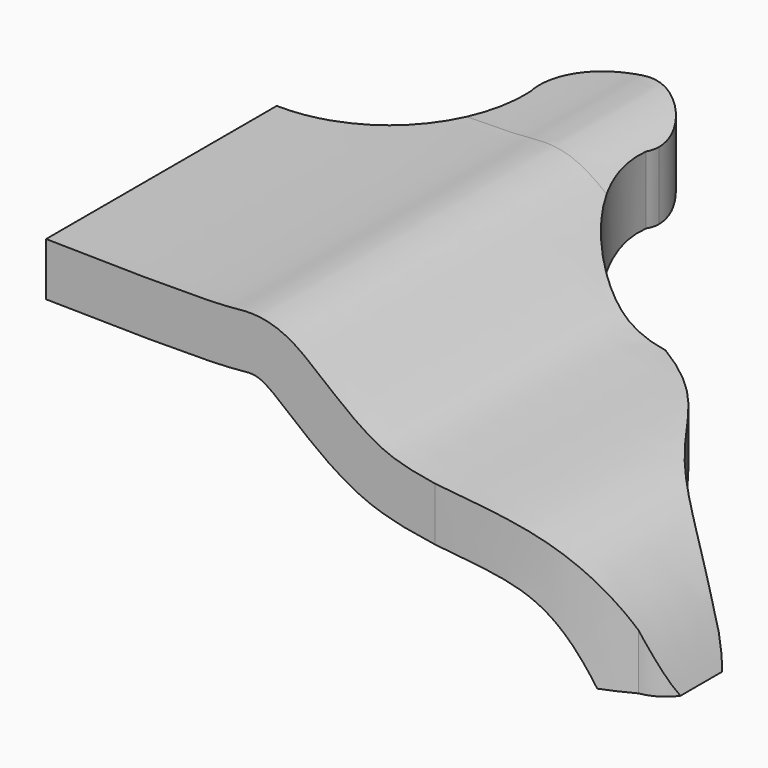
from build123d import *

# Parameters (mm, degrees)
F0_W     = 38.7765130397
F0_H     = 28.7499961852
F1_DEPTH = 25.4
F3_DEPTH = 52.3281


# Not quite as in the source:
# - the dataset's text gives a spline's control points without its knots; the knots are read off the source's solid


with BuildPart() as f1:
    # F0 (on Top) → F1 (new body)
    with BuildSketch(Plane.XY):
        with Locations((-58.5247337142, -22.4215921884)):
            Rectangle(F0_W, F0_H)
        with BuildLine():
            add(Edge.make_bspline(
                [(-20.7452494839, -24.9467859681), (-32.7285714447, -18.2691290975), (-29.7880473778, -12.7225419934), (-39.1364771944, -8.0465940958)],
                knots=[0, 0, 0, 0, 24.9770643195, 24.9770643195, 24.9770643195, 24.9770643195], degree=3))
            Line((-39.1364771944, -8.0465940958), (-39.1364771944, -36.796590281))
            add(Edge.make_bspline(
                [(-21.6266345422, -33.3072070565), (-26.8408916891, -36.1053347588), (-31.1733841196, -36.4459350758), (-39.1364771944, -36.796590281)],
                knots=[0, 0, 0, 0, 17.8541419562, 17.8541419562, 17.8541419562, 17.8541419562], degree=3))
            ThreePointArc((-21.6266345422, -33.3072070565), (-26.6747523502, -28.5483467807), (-20.7452494839, -24.9467859681))
        make_face()
        with BuildLine():
            Line((-77.9129902341, -8.0465940958), (-39.1364771944, -8.0465940958))
            ThreePointArc((-39.1364771944, -8.0465940958), (-48.9563203317, -3.7867576404), (-52.5551873482, 6.2940995685))
            ThreePointArc((-52.5551873482, 6.2940995685), (-58.4554184925, 1.7344119399), (-64.202624171, 6.4855281998))
            ThreePointArc((-64.202624171, 6.4855281998), (-67.9235368456, -3.7375679261), (-77.9129902341, -8.0465940958))
        make_face()
        with BuildLine():
            ThreePointArc((-52.3861701194, 7.7047302995), (-52.4893196056, 7.0016484232), (-52.5551873482, 6.2940995685))
            ThreePointArc((-52.5551873482, 6.2940995685), (-52.428574999, 6.9943702002), (-52.3861701194, 7.7047302995))
        make_face()
        with BuildLine():
            ThreePointArc((-64.202624171, 6.4855281998), (-58.4554184925, 1.7344119399), (-52.5551873482, 6.2940995685))
            ThreePointArc((-52.5551873482, 6.2940995685), (-52.4893196056, 7.0016484232), (-52.3861701194, 7.7047302995))
            ThreePointArc((-52.3861701194, 7.7047302995), (-58.3572947688, 13.6758549489), (-64.3284194183, 7.7047302995))
            ThreePointArc((-64.3284194183, 7.7047302995), (-64.25191384, 7.0965332958), (-64.202624171, 6.4855281998))
        make_face()
        with BuildLine():
            ThreePointArc((-17.9783150406, -29.0054846555), (-18.7358556497, -26.5494227035), (-20.7452494839, -24.9467859681))
            ThreePointArc((-20.7452494839, -24.9467859681), (-26.6747523502, -28.5483467807), (-21.6266345422, -33.3072070565))
            ThreePointArc((-21.6266345422, -33.3072070565), (-19.0132103995, -31.8257262587), (-17.9783150406, -29.0054846555))
        make_face()
        with BuildLine():
            ThreePointArc((-64.3284194183, 7.7047302995), (-64.2968873499, 7.0918930038), (-64.202624171, 6.4855281998))
            ThreePointArc((-64.202624171, 6.4855281998), (-64.25191384, 7.0965332958), (-64.3284194183, 7.7047302995))
        make_face()
    extrude(amount=F1_DEPTH)

    # F2 (on Front) → F3 (intersect, symmetric)
    with BuildSketch(Plane.XZ):
        with BuildLine():
            Line((-83.5097134113, 23.1158043852), (-83.5097134113, 17.8208694641))
            add(Edge.make_bspline(
                [(-83.5097134113, 17.8208694641), (-73.2141432389, 17.6012117472), (-59.4721074922, 17.3165817632), (-56.0034165776, 18.3757243334), (-46.3284903618, 7.642872625), (-29.7396785929, 9.4111190333), (-25.7341444976, 2.4053329313), (-24.2955241086, -0.7361314809)],
                knots=[0.0044584156, 0.0044584156, 0.0044584156, 0.0044584156, 0.2819490011, 0.3784705138, 0.5786724299, 0.805506078, 0.9647305153, 0.9647305153, 0.9647305153, 0.9647305153], degree=3))
            Line((-24.2955241086, -0.7361314809), (-18.5064263501, -0.7361314809))
            add(Edge.make_bspline(
                [(-83.5097134113, 23.1158043852), (-82.4781386863, 23.0937914709), (-80.2903146859, 23.0472099161), (-76.9981774644, 22.9801954036), (-73.6932287125, 22.9197718994), (-70.5558224712, 22.8729918902), (-67.6419029261, 22.8443142653), (-65.0096071237, 22.8380766716), (-63.102389, 22.8549816344), (-61.7850022894, 22.8832373694), (-60.9126200416, 22.9118476507), (-60.2941411796, 22.9415286214), (-59.8740232462, 22.9679855464), (-59.6473632964, 22.9850963908), (-59.4859188095, 22.9990708001), (-59.3198092264, 23.0145236369), (-59.1051961025, 23.0360285686), (-58.8179204127, 23.0652278806), (-58.3739440435, 23.1057107709), (-57.8017054424, 23.1412192711), (-57.0737535882, 23.12250667), (-56.2604305947, 23.0442124599), (-55.3729757598, 22.8456197627), (-54.5424856407, 22.5395884268), (-53.9648791823, 22.2743431246), (-53.436469248, 21.9857184255), (-52.9760804246, 21.7008348435), (-52.5541084992, 21.4160359973), (-52.026466607, 21.0358377149), (-51.4059279542, 20.5556807256), (-50.6800107035, 19.9664629449), (-49.9532373471, 19.3658754398), (-48.9712636304, 18.5585457673), (-47.7109351838, 17.5597718388), (-46.4206563979, 16.6525411456), (-45.3964729568, 16.0300326546), (-44.7676247107, 15.6928429089), (-44.274689501, 15.4578663159), (-43.9144474487, 15.3010634685), (-43.5516274784, 15.1588496563), (-43.0364374651, 14.9771581172), (-42.3464609309, 14.7700291546), (-41.1447324503, 14.4774798421), (-39.4780222241, 14.1796453841), (-37.2743077991, 13.884978231), (-35.3104650042, 13.6294627302), (-33.676270949, 13.3659057937), (-32.419909539, 13.1208960953), (-31.1335029909, 12.807609082), (-29.8177440076, 12.3995053974), (-28.7031198053, 11.9545980284), (-27.8041413297, 11.5154556037), (-26.9193922091, 11.0217097709), (-25.8962646782, 10.3357894381), (-24.7915089535, 9.4220420748), (-23.8108854797, 8.4462482206), (-22.6544914551, 7.0912339426), (-21.4593159075, 5.3419894381), (-20.309325047, 3.2427126697), (-19.3459416873, 1.1940083361), (-18.7794978158, -0.1086191664), (-18.5064263501, -0.7361314809)],
                knots=[0.0034437956, 0.0034437956, 0.0034437956, 0.0034437956, 0.03125, 0.0625, 0.09375, 0.125, 0.15625, 0.1875, 0.21875, 0.234375, 0.25, 0.265625, 0.2734375, 0.28125, 0.28515625, 0.2890625, 0.296875, 0.3046875, 0.3125, 0.328125, 0.3359375, 0.34375, 0.359375, 0.3671875, 0.375, 0.3828125, 0.390625, 0.3984375, 0.40625, 0.421875, 0.4375, 0.453125, 0.46875, 0.5, 0.53125, 0.546875, 0.5625, 0.5703125, 0.578125, 0.5859375, 0.59375, 0.609375, 0.625, 0.65625, 0.6875, 0.71875, 0.734375, 0.75, 0.765625, 0.78125, 0.796875, 0.8046875, 0.8125, 0.828125, 0.84375, 0.859375, 0.875, 0.90625, 0.9375, 0.96875, 1, 1, 1, 1], degree=3))
        make_face()
    extrude(amount=F3_DEPTH, both=True, mode=Mode.INTERSECT)


solid = f1.part
